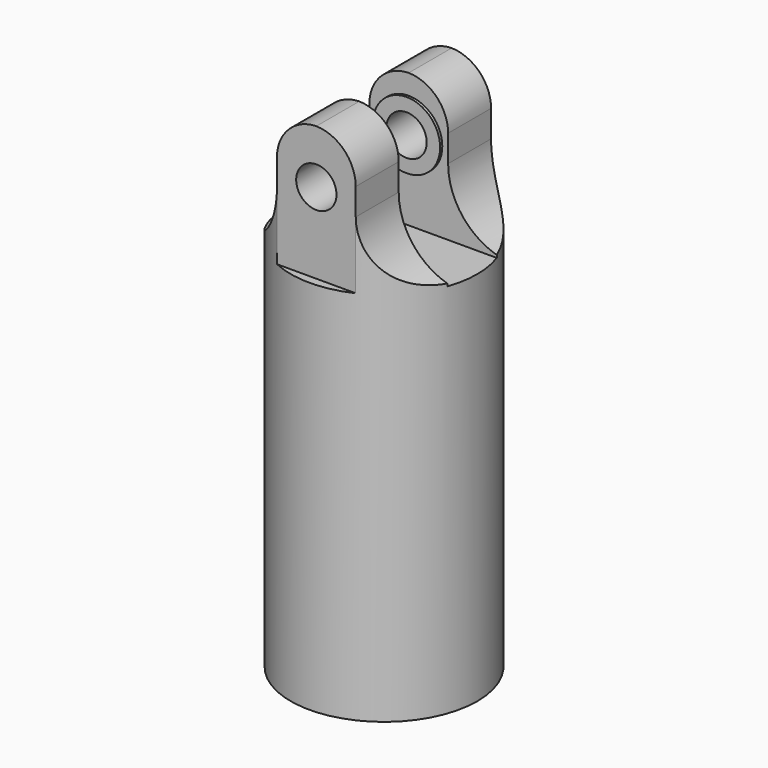
from build123d import *

# Parameters (mm, degrees)
F0_R         = 6.95
F1_DEPTH     = 28
F2_W         = 2.9347061182
F2_H         = 4
F3_DEPTH     = 10
F4_T1_DEPTH  = 19
F4_T3_DEPTH  = 19
F5_T4_DEPTH  = 4
F5_S5_R      = 6.95
F5_T6_DEPTH  = 6
F5_T10_DEPTH = 4
F5_S11_R     = 6.95
F5_T12_DEPTH = 6
F5_T16_DEPTH = 4
F5_S17_R     = 6.95
F5_T18_DEPTH = 6
F5_T22_DEPTH = 4
F5_S23_R     = 6.95
F5_T24_DEPTH = 6
F7_W         = 12.5890113413
F7_H         = 2
F8_DEPTH     = 10
F9_W         = 12.1756089176
F9_H         = 2
F10_DEPTH    = 3
F11_R        = 2.5
F12_DEPTH    = 0.2
F13_R        = 2.5
F14_DEPTH    = 0.2
F15_DEPTH    = 13.2510001


# Not quite as in the source:
# - a fillet or chamfer that OpenCascade refuses, or shapes differently, is made with other operations: its cross-section is extruded or revolved along the edge and cut away or added


with BuildPart() as f1:
    # F0 (on Top) → F1 (new body)
    with BuildSketch(Plane.XY):
        with Locations((-16.023524542, 6.9519880981)):
            Circle(F0_R)
    extrude(amount=F1_DEPTH)

    # F2 (on face) → F3 (join)
    with BuildSketch(Plane.XY.offset(28)):
        with Locations((-17.490877601, 11.2519880981)):
            Rectangle(F2_W, F2_H)
        with Locations((-14.5561714829, 11.2519880981)):
            Rectangle(F2_W, F2_H)
        with Locations((-17.490877601, 2.6519880981)):
            Rectangle(F2_W, F2_H)
        with Locations((-14.5561714829, 2.6519880981)):
            Rectangle(F2_W, F2_H)
    extrude(amount=F3_DEPTH)

    # F4: fillet of radius 3 on 4 edges, made by hand

    # F4_s2 → F4_t1 (cut)
    with BuildSketch(Plane.XZ.offset(-12.1519880981)):
        with BuildLine():
            ThreePointArc((-13.0888184238, 35), (-13.9674980802, 37.1213203436), (-16.0888184238, 38))
            Line((-16.0888184238, 38), (-13.0888184238, 38))
            Line((-13.0888184238, 38), (-13.0888184238, 35))
        make_face()
        with BuildLine():
            ThreePointArc((-18.9582306601, 35), (-18.0795510037, 37.1213203436), (-15.9582306601, 38))
            Line((-15.9582306601, 38), (-18.9582306601, 38))
            Line((-18.9582306601, 38), (-18.9582306601, 35))
        make_face()
    extrude(amount=F4_T1_DEPTH, mode=Mode.SUBTRACT)

    # F4_s4 → F4_t3 (cut)
    with BuildSketch(Plane.XZ.offset(-20.7519880981)):
        with BuildLine():
            ThreePointArc((-13.0888184238, 35), (-13.9674980802, 37.1213203436), (-16.0888184238, 38))
            Line((-16.0888184238, 38), (-13.0888184238, 38))
            Line((-13.0888184238, 38), (-13.0888184238, 35))
        make_face()
        with BuildLine():
            ThreePointArc((-18.9582306601, 35), (-18.0795510037, 37.1213203436), (-15.9582306601, 38))
            Line((-15.9582306601, 38), (-18.9582306601, 38))
            Line((-18.9582306601, 38), (-18.9582306601, 35))
        make_face()
    extrude(amount=F4_T3_DEPTH, mode=Mode.SUBTRACT)

    # F5: fillet of radius 5 on 4 edges, made by hand


with BuildPart() as f5_tool2:
    # F5_s3 → F5_t4 (new body)
    with BuildSketch(Plane.XZ.offset(-0.6519880981)):
        with BuildLine():
            ThreePointArc((-13.0888184238, 33), (-11.6243523297, 29.4644660941), (-8.0888184238, 28))
            Line((-8.0888184238, 28), (-8.0888184238, 27.9))
            Line((-8.0888184238, 27.9), (-13.1888184238, 27.9))
            Line((-13.1888184238, 27.9), (-13.1888184238, 33))
            Line((-13.1888184238, 33), (-13.0888184238, 33))
        make_face()
    extrude(amount=-F5_T4_DEPTH)

    # F5_s5 → F5_t6 (intersect, symmetric)
    with BuildSketch(Plane.XY.offset(30.4)):
        with Locations((-16.023524542, 6.9519880981)):
            Circle(F5_S5_R)
    extrude(amount=F5_T6_DEPTH, both=True, mode=Mode.INTERSECT)


with BuildPart() as f1_1:
    add(f1.part)

    # F5_t1: union F5_tool2
    add(f5_tool2.part)


with BuildPart() as f5_tool8:
    # F5_s9 → F5_t10 (new body)
    with BuildSketch(Plane.XZ.offset(-9.2519880981)):
        with BuildLine():
            ThreePointArc((-13.0888184238, 33), (-11.6243523297, 29.4644660941), (-8.0888184238, 28))
            Line((-8.0888184238, 28), (-8.0888184238, 27.9))
            Line((-8.0888184238, 27.9), (-13.1888184238, 27.9))
            Line((-13.1888184238, 27.9), (-13.1888184238, 33))
            Line((-13.1888184238, 33), (-13.0888184238, 33))
        make_face()
    extrude(amount=-F5_T10_DEPTH)

    # F5_s11 → F5_t12 (intersect, symmetric)
    with BuildSketch(Plane.XY.offset(30.4)):
        with Locations((-16.023524542, 6.9519880981)):
            Circle(F5_S11_R)
    extrude(amount=F5_T12_DEPTH, both=True, mode=Mode.INTERSECT)


with BuildPart() as f1_2:
    add(f1_1.part)

    # F5_t7: union F5_tool8
    add(f5_tool8.part)


with BuildPart() as f5_tool14:
    # F5_s15 → F5_t16 (new body)
    with BuildSketch(Plane.XZ.offset(-13.2519880981)):
        with BuildLine():
            ThreePointArc((-18.9582306601, 33), (-20.4226967542, 29.4644660941), (-23.9582306601, 28))
            Line((-23.9582306601, 28), (-23.9582306601, 27.9))
            Line((-23.9582306601, 27.9), (-18.8582306601, 27.9))
            Line((-18.8582306601, 27.9), (-18.8582306601, 33))
            Line((-18.8582306601, 33), (-18.9582306601, 33))
        make_face()
    extrude(amount=F5_T16_DEPTH)

    # F5_s17 → F5_t18 (intersect, symmetric)
    with BuildSketch(Plane.XY.offset(30.4)):
        with Locations((-16.023524542, 6.9519880981)):
            Circle(F5_S17_R)
    extrude(amount=F5_T18_DEPTH, both=True, mode=Mode.INTERSECT)


with BuildPart() as f1_3:
    add(f1_2.part)

    # F5_t13: union F5_tool14
    add(f5_tool14.part)


with BuildPart() as f5_tool20:
    # F5_s21 → F5_t22 (new body)
    with BuildSketch(Plane.XZ.offset(-4.6519880981)):
        with BuildLine():
            ThreePointArc((-18.9582306601, 33), (-20.4226967542, 29.4644660941), (-23.9582306601, 28))
            Line((-23.9582306601, 28), (-23.9582306601, 27.9))
            Line((-23.9582306601, 27.9), (-18.8582306601, 27.9))
            Line((-18.8582306601, 27.9), (-18.8582306601, 33))
            Line((-18.8582306601, 33), (-18.9582306601, 33))
        make_face()
    extrude(amount=F5_T22_DEPTH)

    # F5_s23 → F5_t24 (intersect, symmetric)
    with BuildSketch(Plane.XY.offset(30.4)):
        with Locations((-16.023524542, 6.9519880981)):
            Circle(F5_S23_R)
    extrude(amount=F5_T24_DEPTH, both=True, mode=Mode.INTERSECT)


with BuildPart() as f1_4:
    add(f1_3.part)

    # F5_t19: union F5_tool20
    add(f5_tool20.part)

    # F7 (on face) → F8 (cut)
    with BuildSketch(Plane(origin=(0, 0, 0), x_dir=(1, 0, 0), z_dir=(0, 0, -1))):
        with Locations((-17.0201025903, -6.9519880981)):
            Rectangle(F7_W, F7_H)
    extrude(amount=-F8_DEPTH, mode=Mode.SUBTRACT)

    # F11 (on face) → F12 (join)
    with BuildSketch(Plane(origin=(0, 4.6519880981, 0), x_dir=(-1, 0, 0), z_dir=(0, 1, 0))):
        with Locations((16.023524542, 34)):
            Circle(F11_R)
    extrude(amount=F12_DEPTH)

    # F13 (on face) → F14 (join)
    with BuildSketch(Plane.XZ.offset(-9.2519880981)):
        with Locations((-16.023524542, 34)):
            Circle(F13_R)
    extrude(amount=F14_DEPTH)

    # F6 (on face) → F15 (cut, through all)
    with BuildSketch(Plane(origin=(0, 13.2519880981, 0), x_dir=(-1, 0, 0), z_dir=(0, 1, 0))):
        with BuildLine():
            ThreePointArc((17.523524542, 34), (16.023524542, 35.5), (14.523524542, 34))
            Line((14.523524542, 34), (17.523524542, 34))
        make_face()
        with BuildLine():
            Line((17.523524542, 34), (14.523524542, 34))
            ThreePointArc((14.523524542, 34), (16.023524542, 32.5), (17.523524542, 34))
        make_face()
    extrude(amount=-F15_DEPTH, mode=Mode.SUBTRACT)


with BuildPart() as f10:
    # F9 (on face) → F10 (new body)
    with BuildSketch(Plane(origin=(0, 0, 0), x_dir=(1, 0, 0), z_dir=(0, 0, -1))):
        with Locations((-16.8134013785, -6.9519880981)):
            Rectangle(F9_W, F9_H)
    extrude(amount=-F10_DEPTH)


solid = Compound([f1_4.part, f10.part])
